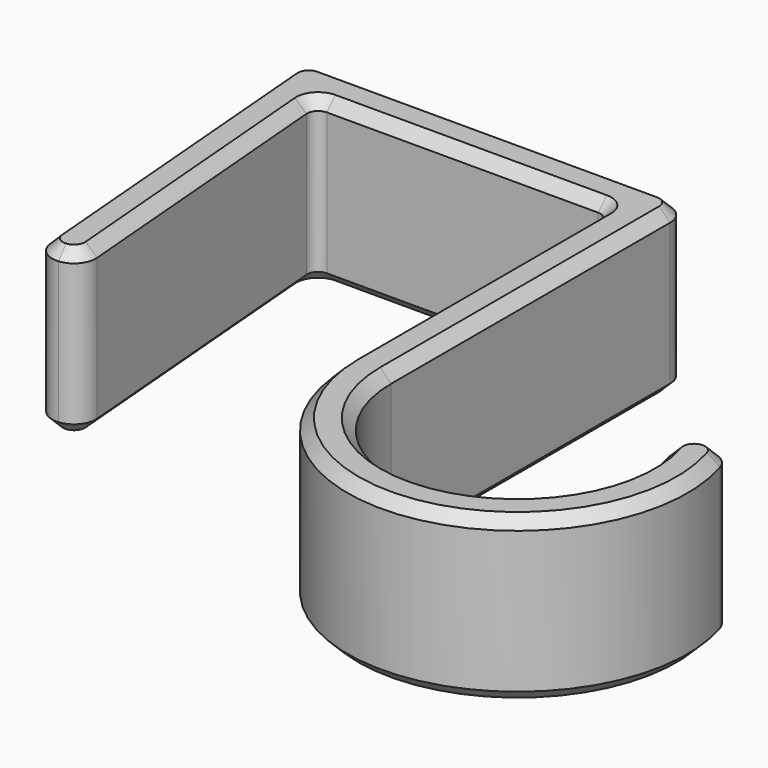
from build123d import *

# Parameters (mm, degrees)
F1_DEPTH = 15
F2_R     = 1.99999
F3_R     = 2
F4_R     = 1
F5_SIZE  = 1


# Not quite as in the source:
# - a fillet or chamfer is up to 0.001 mm smaller than in the source, because OpenCascade refuses the exact size


with BuildPart() as f1:
    # F0 (on Top) → F1 (new body)
    with BuildSketch(Plane.XY):
        with BuildLine():
            Line((2.5, -29.8956518578), (0, 0))
            Line((0, 0), (27, 0))
            Line((27, 0), (27, -30))
            ThreePointArc((27, -30), (45.6594117082, -45.2970585408), (57, -24))
            Line((57, -24), (52.5277389168, -24))
            ThreePointArc((52.5277389168, -24), (45.7143401039, -41.1741167757), (31, -30))
            Line((31, -30), (31, 4))
            Line((31, 4), (-4.348458452, 4))
            Line((-4.348458452, 4), (-1.4860869144, -30.2289851911))
            Line((-1.4860869144, -30.2289851911), (2.5, -29.8956518578))
        make_face()
    extrude(amount=F1_DEPTH)

    # F2 (radius 2 in the source; OpenCascade refuses exactly that, so slightly less here)
    f2_edges = [f1.edges().sort_by_distance(p)[0] for p in [
        (2.5, -29.895652, 7.5),
        (-1.486087, -30.228985, 7.5),
        (52.527739, -24, 7.5),
        (57, -24, 7.5),
    ]]
    fillet(f2_edges, radius=F2_R)

    # F3
    f3_edges = [f1.edges().sort_by_distance(p)[0] for p in [
        (31, 4, 7.5),
        (-4.348458, 4, 7.5),
    ]]
    fillet(f3_edges, radius=F3_R)

    # F4
    f4_edges = [f1.edges().sort_by_distance(p)[0] for p in [
        (0, 0, 7.5),
        (27, 0, 7.5),
    ]]
    fillet(f4_edges, radius=F4_R)

    # F5
    f5_edges = [f1.edges().sort_by_distance(p)[0] for p in [
        (1.211964, -14.492976, 15),
        (0.351135, -0.322997, 15),
        (1.867439, -29.360721, 15),
        (13.543557, 0, 15),
        (0.506957, -30.062319, 15),
        (26.707107, -0.292893, 15),
        (-0.951156, -29.596424, 15),
        (27, -15.5, 15),
        (-2.910013, -13.201309, 15),
        (44.919918, -45.426535, 15),
        (-3.646189, 3.354006, 15),
        (56.78664, -24.391198, 15),
        (13.412885, 4, 15),
        (55.598458, -24, 15),
        (30.414214, 3.414214, 15),
        (53.989656, -24.81182, 15),
        (31, -14, 15),
        (44.32507, -41.471013, 15),
        (1.211964, -14.492976, 0),
        (0.351135, -0.322997, 0),
        (1.867439, -29.360721, 0),
        (13.543557, 0, 0),
        (0.506957, -30.062319, 0),
        (26.707107, -0.292893, 0),
        (-0.951156, -29.596424, 0),
        (27, -15.5, 0),
        (-2.910013, -13.201309, 0),
        (44.919918, -45.426535, 0),
        (-3.646189, 3.354006, 0),
        (56.78664, -24.391198, 0),
        (13.412885, 4, 0),
        (55.598458, -24, 0),
        (30.414214, 3.414214, 0),
        (53.989656, -24.81182, 0),
        (31, -14, 0),
        (44.32507, -41.471013, 0),
    ]]
    chamfer(f5_edges, length=F5_SIZE)


solid = f1.part
